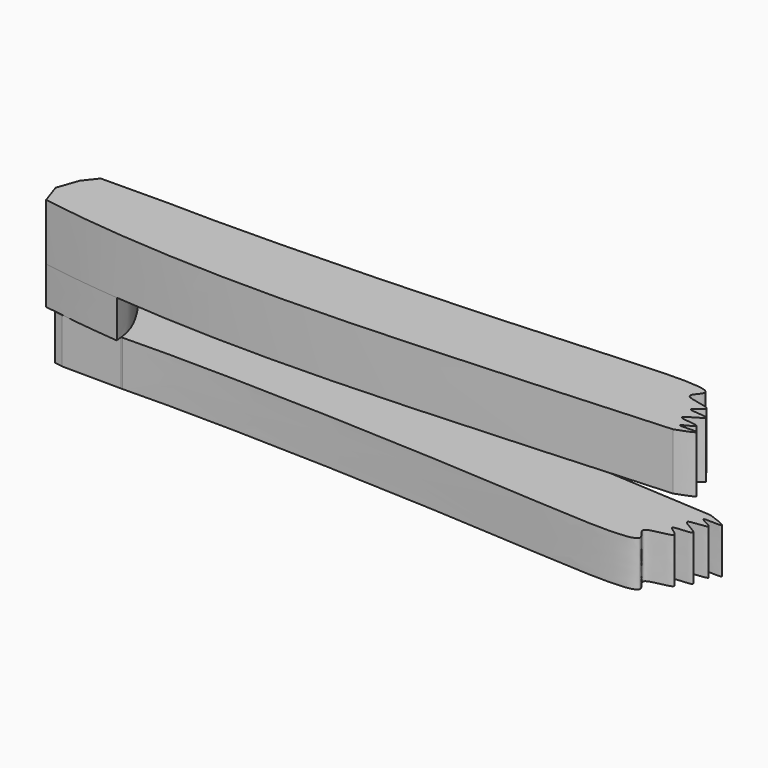
from build123d import *

# Parameters (mm, degrees)
F1_DEPTH = 7.62
F3_DEPTH = 5.08
F5_DEPTH = 6.096


with BuildPart() as f1:
    # F0 (on Top) → F1 (new body)
    with BuildSketch(Plane.XY):
        with BuildLine():
            Line((-32.1232994972, -4.6074000446), (-31.1663517222, -7.402031539))
            add(Edge.make_bspline(
                [(-31.1663517222, -7.402031539), (-24.3620805414, -8.516586495), (-5.1188000961, -10.1180637513), (23.5489427366, -8.8323068142), (43.4879123536, -7.5996602354), (53.0083630423, -7.0088685962)],
                knots=[0.6412967297, 0.6412967297, 0.6412967297, 0.6412967297, 0.7293718882, 0.8688213456, 0.9965033878, 0.9965033878, 0.9965033878, 0.9965033878], degree=3))
            add(Edge.make_bspline(
                [(-20.5886847274, 0.0714136867), (-18.4325246492, 0.0085905521), (-2.904384168, -0.0903390189), (28.4431286792, 1.2110854268), (53.3450981726, 3.225027955), (48.0643964884, -0.5269030489), (54.671286243, -0.6815816974), (49.990725038, -2.7091281295), (56.2250035708, -2.2744194982), (49.8425443069, -4.7372453658), (56.2477520114, -4.4882263671), (51.3064623402, -6.2296941136), (56.9532836508, -5.5567427397), (54.34598679, -6.5234124491), (53.0083630423, -7.0088685962)],
                knots=[0.4762517442, 0.4762517442, 0.4762517442, 0.4762517442, 0.4999643977, 0.6391192862, 0.7242199913, 0.7509257777, 0.7881752399, 0.8140897202, 0.8458528044, 0.8781751537, 0.9100717752, 0.9367812247, 0.9676122856, 1, 1, 1, 1], degree=3))
            Line((-20.5886847274, 0.0714136867), (-29.733825475, 0))
            Line((-29.733825475, 0), (-31.1305152205, -1.7574477268))
            Line((-31.1305152205, -1.7574477268), (-32.1232994972, -4.6074000446))
        make_face()
    extrude(amount=F1_DEPTH)

    # F2 (on face) → F3 (join)
    with BuildSketch(Plane(origin=(0, 0, 0), x_dir=(1, 0, 0), z_dir=(0, 0, -1))):
        with BuildLine():
            Line((-31.1663517222, 7.402031539), (-32.1232994972, 4.6074000446))
            Line((-32.1232994972, 4.6074000446), (-31.3824697288, 2.4807250306))
            add(Edge.make_bspline(
                [(-28.9687315599, -0.0059745584), (-30.1065744803, 0.5836866376), (-30.8737077287, 1.5004076818), (-31.3824697288, 2.4807250306)],
                knots=[0.4887841261, 0.4887841261, 0.4887841261, 0.4887841261, 0.5523463493, 0.5523463493, 0.5523463493, 0.5523463493], degree=3))
            Line((-28.9687315599, -0.0059745584), (-24.5685748837, -0.0403350367))
            add(Edge.make_bspline(
                [(-20.5886847274, 8.7179279132), (-20.6959150874, 7.6662220966), (-20.9405487627, 5.2668768071), (-23.2119366173, 1.8933456436), (-24.5685748837, -0.0403350367)],
                knots=[0, 0, 0, 0, 0.4053640786, 0.924791303, 0.924791303, 0.924791303, 0.924791303], degree=3))
            add(Edge.make_bspline(
                [(-31.1663517222, 7.402031539), (-27.768990322, 7.9585269939), (-24.2108723521, 8.3917141444), (-20.5886847274, 8.7179279132)],
                knots=[0.6412967297, 0.6412967297, 0.6412967297, 0.6412967297, 0.6852725114, 0.6852725114, 0.6852725114, 0.6852725114], degree=3))
        make_face()
    extrude(amount=F3_DEPTH)


with BuildPart() as f5:
    # F4 (on face) → F5 (new body)
    with BuildSketch(Plane(origin=(0, 0, -5.08), x_dir=(1, 0, 0), z_dir=(0, 0, -1))):
        with BuildLine():
            add(Edge.make_bspline(
                [(-29.0925031999, 0.0602487535), (-30.1625283777, 0.6510527228), (-30.8923773853, 1.5363816503), (-31.3824697288, 2.4807250306)],
                knots=[0.4911166212, 0.4911166212, 0.4911166212, 0.4911166212, 0.5523463493, 0.5523463493, 0.5523463493, 0.5523463493], degree=3))
            add(Edge.make_bspline(
                [(-29.0925031999, 0.0602487535), (-28.9346911942, 0.0370119911), (-28.776583455, 0.0140256194), (-28.6181891843, -0.0087119163)],
                knots=[0.6498872135, 0.6498872135, 0.6498872135, 0.6498872135, 0.6518950105, 0.6518950105, 0.6518950105, 0.6518950105], degree=3))
            Line((-28.6181891843, -0.0087119163), (-24.5685748837, -0.0403350367))
            add(Edge.make_bspline(
                [(-20.685481243, 7.8445616496), (-20.7845843132, 7.0723755723), (-21.2149092951, 4.8593885816), (-23.2119366173, 1.8933456436), (-24.5685748837, -0.0403350367)],
                knots=[0.111705376, 0.111705376, 0.111705376, 0.111705376, 0.4053640786, 0.924791303, 0.924791303, 0.924791303, 0.924791303], degree=3))
            Line((-20.685481243, 7.8445616496), (-28.6908726534, 7.782048176))
            add(Edge.make_bspline(
                [(-29.7920200182, 7.619164839), (-29.4266012407, 7.6748204882), (-29.059513444, 7.7291083999), (-28.6908726534, 7.782048176)],
                knots=[0.6471901897, 0.6471901897, 0.6471901897, 0.6471901897, 0.6518633268, 0.6518633268, 0.6518633268, 0.6518633268], degree=3))
            Line((-29.7920200182, 7.619164839), (-31.0653300909, 6.016965138))
            Line((-31.0653300909, 6.016965138), (-31.8398266317, 3.7936440565))
            Line((-31.8398266317, 3.7936440565), (-31.3824697288, 2.4807250306))
        make_face()
        with BuildLine():
            Line((-24.5685748837, -0.0403350367), (-28.6181891843, -0.0087119163))
            add(Edge.make_bspline(
                [(-28.6181891843, -0.0087119163), (-22.5060705197, -0.8861080217), (-4.1982571595, -2.3052878302), (23.6141278662, -1.0578939494), (43.5530974832, 0.1747526294), (53.0735481719, 0.7655442686)],
                knots=[0.6518950105, 0.6518950105, 0.6518950105, 0.6518950105, 0.7293718882, 0.8688213456, 0.9965033878, 0.9965033878, 0.9965033878, 0.9965033878], degree=3))
            add(Edge.make_bspline(
                [(-20.5234995978, 7.8458265515), (-18.3673395195, 7.7830034169), (-2.8391990384, 7.6840738459), (28.5083138088, 8.9854982916), (53.4102833022, 10.9994408198), (48.129581618, 7.2475098159), (54.7364713727, 7.0928311674), (50.0559101676, 5.0652847353), (56.2901887005, 5.4999933666), (49.9077294366, 3.037167499), (56.3129371411, 3.2861864977), (51.3716474698, 1.5447187512), (57.0184687805, 2.2176701251), (54.4111719196, 1.2510004157), (53.0735481719, 0.7655442686)],
                knots=[0.4762517442, 0.4762517442, 0.4762517442, 0.4762517442, 0.4999643977, 0.6391192862, 0.7242199913, 0.7509257777, 0.7881752399, 0.8140897202, 0.8458528044, 0.8781751537, 0.9100717752, 0.9367812247, 0.9676122856, 1, 1, 1, 1], degree=3))
            Line((-20.5234995978, 7.8458265515), (-20.685481243, 7.8445616496))
            add(Edge.make_bspline(
                [(-20.685481243, 7.8445616496), (-20.7845843132, 7.0723755723), (-21.2149092951, 4.8593885816), (-23.2119366173, 1.8933456436), (-24.5685748837, -0.0403350367)],
                knots=[0.111705376, 0.111705376, 0.111705376, 0.111705376, 0.4053640786, 0.924791303, 0.924791303, 0.924791303, 0.924791303], degree=3))
        make_face()
    extrude(amount=F5_DEPTH)


solid = Compound([f1.part, f5.part])
